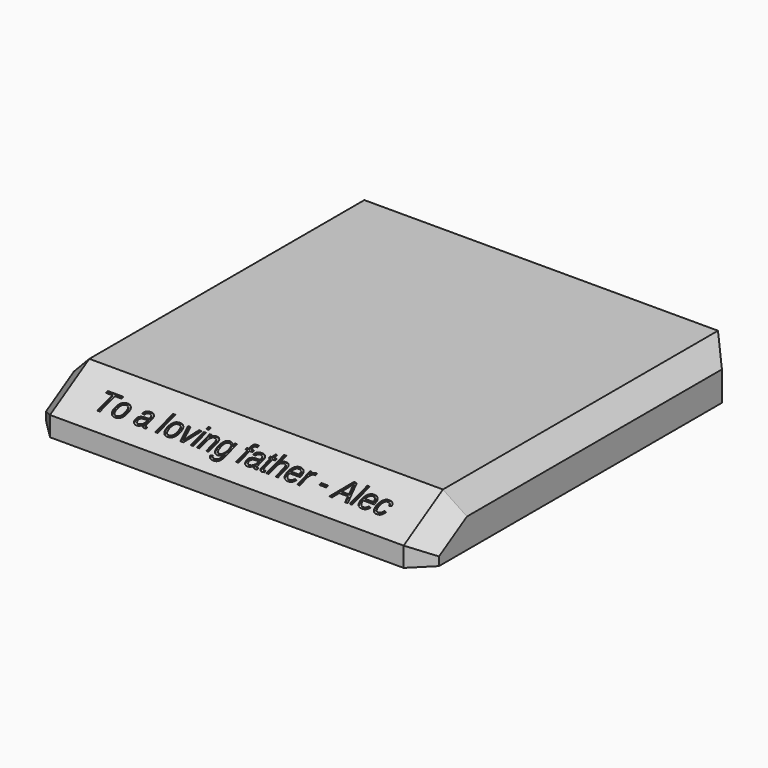
from build123d import *

# Parameters (mm, degrees)
F0_W         = 101.6
F0_H         = 101.6
F1_DEPTH     = 12.7
F2_SIZE2     = 12.7
F2_SIZE      = 7.62
F3_SIZE      = 5.08
F4_TEXT_SIZE = 7.1765138695
F5_DEPTH     = 0.3048


# Not quite as in the source:
# - Text() gives the source's letters only with a copy of the font that has no kerning and outlines rounded to 1/6400 em; it was checked with that copy


with BuildPart() as f1:
    # F0 (on Top) → F1 (new body)
    with BuildSketch(Plane.XY):
        Rectangle(F0_W, F0_H)
    extrude(amount=F1_DEPTH)

    # F2
    f2_edges = [f1.edges().sort_by_distance(p)[0] for p in [
        (0, -50.8, 12.7),
    ]]
    f2_side = f1.faces().sort_by_distance((0, -50.8, 6.35))[0]
    chamfer(f2_edges, length=F2_SIZE, length2=F2_SIZE2, reference=f2_side)

    # F3
    f3_edges = [f1.edges().sort_by_distance(p)[0] for p in [
        (-50.8, -50.8, 2.54),
        (-50.8, -44.45, 8.89),
        (-50.8, 6.35, 12.7),
        (50.8, -50.8, 2.54),
        (50.8, -44.45, 8.89),
        (50.8, 6.35, 12.7),
        (50.8, 50.8, 6.35),
        (-50.8, 50.8, 6.35),
    ]]
    chamfer(f3_edges, length=F3_SIZE)

    # F4 (on face) → F5 (cut)
    with BuildSketch(Plane(origin=(0, -15.6882352941, 26.1470588235), x_dir=(1, 0, 0), z_dir=(0, -0.5144957554, 0.8574929257))):
        with Locations((-38.1, -36.3834761083)):
            Text('To a loving father - Alec', F4_TEXT_SIZE, font='Arimo', font_style=FontStyle.ITALIC, text_align=(TextAlign.LEFT, TextAlign.BOTTOM))
    extrude(amount=-F5_DEPTH, mode=Mode.SUBTRACT)


solid = f1.part
